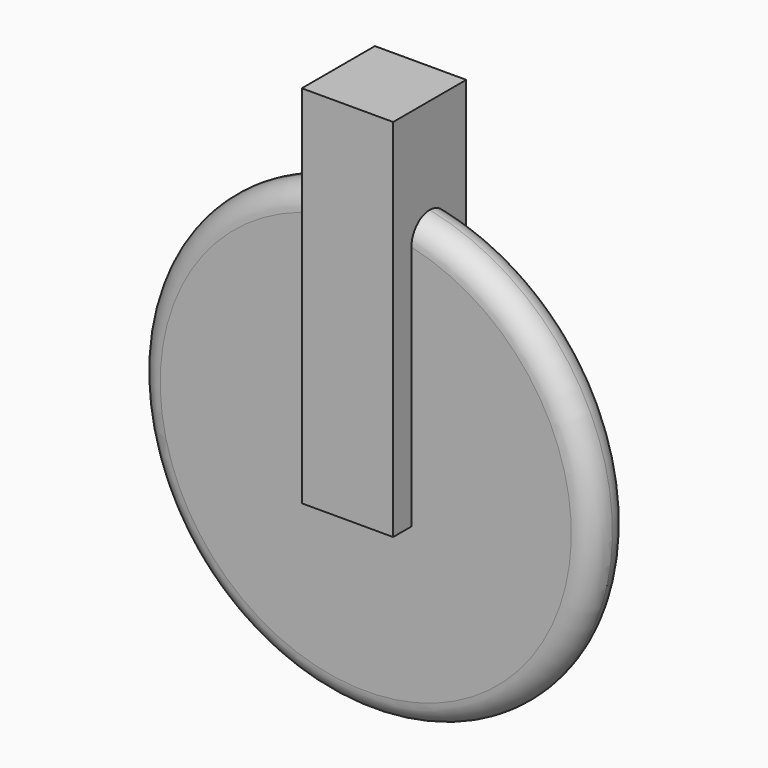
from build123d import *

# Parameters (mm, degrees)
F0_R     = 63.5
F0_R_2   = 6.35
F1_DEPTH = 6.35
F2_R     = 6.34999
F4_DEPTH = 12.7


# Not quite as in the source:
# - a fillet or chamfer is up to 0.001 mm smaller than in the source, because OpenCascade refuses the exact size


with BuildPart() as f1:
    # F0 (on Front) → F1 (new body, symmetric)
    with BuildSketch(Plane.XZ):
        Circle(F0_R)
        Circle(F0_R_2, mode=Mode.SUBTRACT)
    extrude(amount=F1_DEPTH, both=True)

    # F2 (radius 6.35 in the source; OpenCascade refuses exactly that, so slightly less here)
    f2_edges = [f1.edges().sort_by_distance(p)[0] for p in [
        (-63.5, -6.35, 0),
        (-63.5, 6.35, 0),
    ]]
    fillet(f2_edges, radius=F2_R)

    # F3 (on Right) → F4 (join, symmetric)
    with BuildSketch(Plane.YZ):
        Polygon((-12.7, -12.7), (0, -12.7), (12.7, -12.7), (12.7, 88.9), (-12.7, 88.9), align=None)
    extrude(amount=F4_DEPTH, both=True)


solid = f1.part
